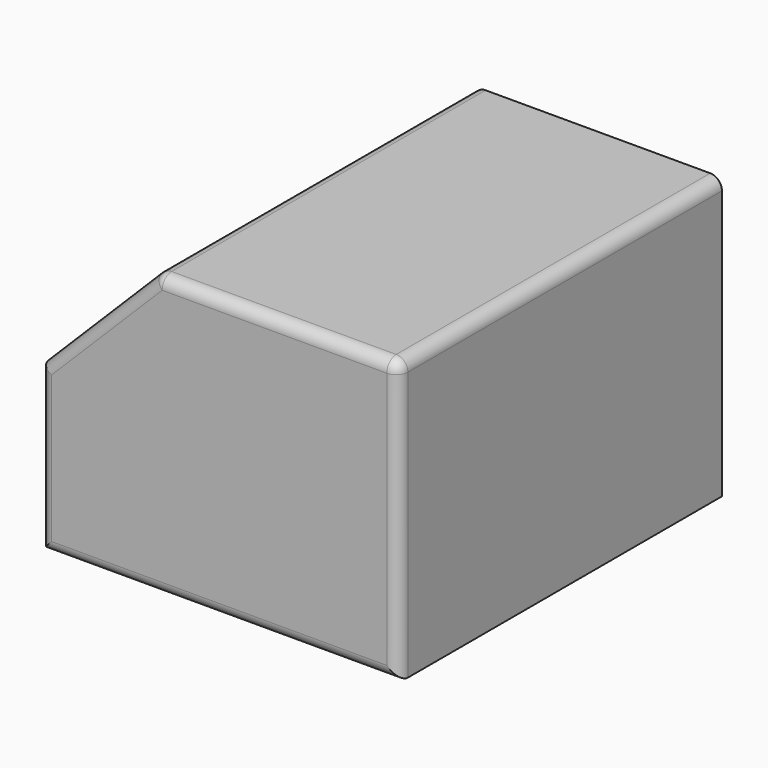
from build123d import *

# Parameters (mm, degrees)
F0_W         = 155.1840901375
F0_H         = 121.4890033007
F1_DEPTH     = 174.9801635742
F2_SIZE      = 50.8
F3_R         = 5.08
F4_T1_DEPTH  = 182.6001635742
F4_T3_DEPTH  = 175.1606758164
F4_T8_DEPTH  = 5.08
F4_S13_W     = 5.08
F4_S13_H     = 5.08
F4_T14_DEPTH = 5.08


# Not quite as in the source:
# - a fillet or chamfer that OpenCascade refuses, or shapes differently, is made with other operations: its cross-section is extruded or revolved along the edge and cut away or added


with BuildPart() as f1:
    # F0 (on Front) → F1 (new body)
    with BuildSketch(Plane.XZ):
        with Locations((77.5920450687, 60.7445016503)):
            Rectangle(F0_W, F0_H)
    extrude(amount=F1_DEPTH)

    # F2
    f2_edges = [f1.edges().sort_by_distance(p)[0] for p in [
        (0, -87.490082, 121.489003),
    ]]
    chamfer(f2_edges, length=F2_SIZE)

    # F3
    f3_edges = [f1.edges().sort_by_distance(p)[0] for p in [
        (25.4, -174.980164, 96.089003),
        (0, -174.980164, 35.344502),
        (77.592045, -174.980164, 0),
        (102.992045, -174.980164, 121.489003),
        (155.18409, -174.980164, 60.744502),
    ]]
    fillet(f3_edges, radius=F3_R)

    # F4: fillet of radius 5.08 on 4 edges, made by hand

    # F4_s2 → F4_t1 (cut)
    with BuildSketch(Plane.XZ.offset(-12.7)):
        with BuildLine():
            ThreePointArc((150.1040901375, 121.4890033007), (153.6961925859, 120.0011057491), (155.1840901375, 116.4090033007))
            Line((155.1840901375, 116.4090033007), (155.1840901375, 121.4890033007))
            Line((155.1840901375, 121.4890033007), (150.1040901375, 121.4890033007))
        make_face()
    extrude(amount=F4_T1_DEPTH, mode=Mode.SUBTRACT)

    # F4_s4 → F4_t3 (cut)
    with BuildSketch(Plane.XZ.offset(-5.2605122421)):
        with BuildLine():
            ThreePointArc((49.3121024484, 120.0011057491), (50.9601730604, 121.1023113258), (52.9042048969, 121.4890033007))
            Line((52.9042048969, 121.4890033007), (50.8, 121.4890033007))
            Line((50.8, 121.4890033007), (49.3121024484, 120.0011057491))
        make_face()
    extrude(amount=F4_T3_DEPTH, mode=Mode.SUBTRACT)


with BuildPart() as f4_tool6:
    # F4_s7 → F4_t8 (new body)
    with BuildSketch(Plane.XZ.offset(169.9001635742)):
        Polygon((52.9042048969, 116.4090033007), (49.3121024484, 120.0011057491), (50.8, 121.4890033007), (52.9042048969, 121.4890033007), align=None)
    extrude(amount=F4_T8_DEPTH)

    # F4_s9 → F4_t10 (revolve, cut)
    with BuildSketch(Plane(origin=(52.9042048969, -169.9001635742, 116.4090033007), x_dir=(0.3826834324, 0, -0.9238795325), z_dir=(-0.9238795325, 0, -0.3826834324))):
        with BuildLine():
            ThreePointArc((0, -5.08), (5.08, 0), (0, 5.08))
            Line((0, 5.08), (0, -5.08))
        make_face()
    revolve(axis=Axis((52.9042048969, -169.9001635742, 116.4090033007), (0, -1, 0)), mode=Mode.SUBTRACT)


with BuildPart() as f1_1:
    add(f1.part)

    # F4_t5: cut F4_tool6
    add(f4_tool6.part, mode=Mode.SUBTRACT)


with BuildPart() as f4_tool12:
    # F4_s13 → F4_t14 (new body)
    with BuildSketch(Plane.XY.offset(116.4090033007)):
        with Locations((152.6440901375, -172.4401635742)):
            Rectangle(F4_S13_W, F4_S13_H)
    extrude(amount=F4_T14_DEPTH)

    # F4_s15 → F4_t16 (revolve, cut)
    with BuildSketch(Plane(origin=(150.1040901375, -169.9001635742, 116.4090033007), x_dir=(-0.7071067812, 0.7071067812, 0), z_dir=(0.7071067812, 0.7071067812, 0))):
        with BuildLine():
            ThreePointArc((0, -5.08), (5.08, 0), (0, 5.08))
            Line((0, 5.08), (0, -5.08))
        make_face()
    revolve(axis=Axis((150.1040901375, -169.9001635742, 116.4090033007), (0, 0, 1)), mode=Mode.SUBTRACT)


with BuildPart() as f1_2:
    add(f1_1.part)

    # F4_t11: cut F4_tool12
    add(f4_tool12.part, mode=Mode.SUBTRACT)


solid = f1_2.part
